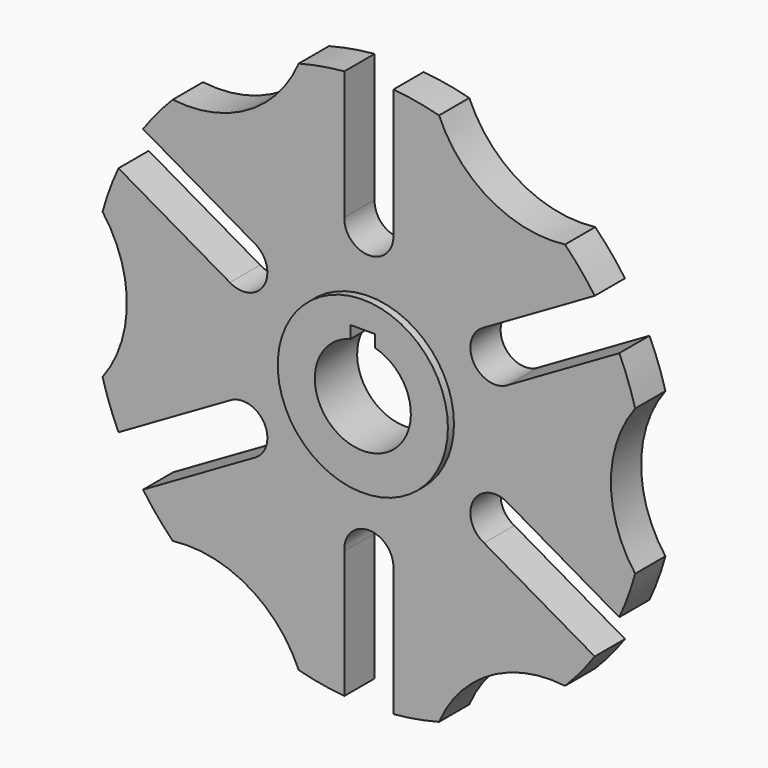
from build123d import *

# Parameters (mm, degrees)
F0_R            = 73
F2_DEPTH        = 5
F4_DEPTH        = 5.001
F4_DEPTH_BACK   = 5.001
F4_COPIES_COUNT = 6
F5_R            = 32
F6_DEPTH        = 5.001
F6_DEPTH_BACK   = 5.001
F6_COPIES_COUNT = 6
F7_R            = 22.5
F8_DEPTH        = 7
F10_DEPTH       = 7.001
F10_DEPTH_BACK  = 7.001


# Not quite as in the source:
# - a pattern or mirror of a feature is missing from the dataset's text; its kind, count and spacing are read off the source's solid


with BuildPart() as f2:
    # F0 (on Front) → F2 (new body, symmetric)
    with BuildSketch(Plane.XZ):
        Circle(F0_R)
    extrude(amount=F2_DEPTH, both=True)

    # F3 (on Front) → F4 (cut, two sides)
    with BuildSketch(Plane.XZ) as f4_sk:
        with BuildLine():
            Line((-6.4973653699, 78.4645676613), (-6.4973653699, 38.6850493181))
            ThreePointArc((-6.4973653699, 38.6850493181), (0.119478264, 32.001098174), (6.4861730913, 38.9237435893))
            Line((6.4861730913, 38.9237435893), (6.4861730913, 78.4645676613))
            Line((6.4861730913, 78.4645676613), (-6.4973653699, 78.4645676613))
        make_face()
    f4 = extrude(amount=-F4_DEPTH, mode=Mode.SUBTRACT) + extrude(f4_sk.sketch, amount=F4_DEPTH_BACK, mode=Mode.SUBTRACT)

    # F4_copies: F4 ×6 about axis
    f4_copies_axis = Axis((0, 0, 0), (0, 1, 0))
    for i in range(1, F4_COPIES_COUNT):
        add(f4.rotate(f4_copies_axis, i * 360 / F4_COPIES_COUNT), mode=Mode.SUBTRACT)

    # F5 (on Front) → F6 (cut, two sides)
    with BuildSketch(Plane.XZ) as f6_sk:
        with Locations((48, 83.1384387633)):
            Circle(F5_R)
    f6 = extrude(amount=-F6_DEPTH, mode=Mode.SUBTRACT) + extrude(f6_sk.sketch, amount=F6_DEPTH_BACK, mode=Mode.SUBTRACT)

    # F6_copies: F6 ×6 about axis
    f6_copies_axis = Axis((0, 0, 0), (0, 1, 0))
    for i in range(1, F6_COPIES_COUNT):
        add(f6.rotate(f6_copies_axis, i * 360 / F6_COPIES_COUNT), mode=Mode.SUBTRACT)

    # F7 (on Front) → F8 (join, symmetric)
    with BuildSketch(Plane.XZ):
        Circle(F7_R)
    extrude(amount=F8_DEPTH, both=True)

    # F9 (on Front) → F10 (cut, two sides)
    with BuildSketch(Plane.XZ) as f10_sk:
        with BuildLine():
            Line((-3.25, 15.5271128528), (-3.25, 12.2771128528))
            ThreePointArc((-3.25, 12.2771128528), (0, -12.7), (3.25, 12.2771128528))
            Line((3.25, 12.2771128528), (3.25, 15.5271128528))
            Line((3.25, 15.5271128528), (-3.25, 15.5271128528))
        make_face()
    extrude(amount=-F10_DEPTH, mode=Mode.SUBTRACT)
    extrude(f10_sk.sketch, amount=F10_DEPTH_BACK, mode=Mode.SUBTRACT)


solid = f2.part
